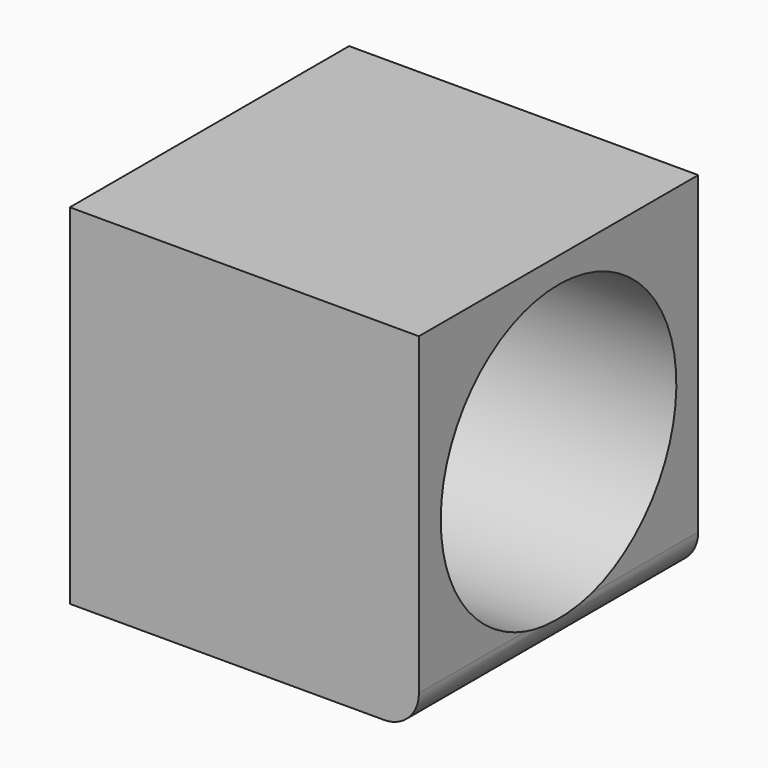
from build123d import *

# Parameters (mm, degrees)
F0_W        = 50
F0_H        = 50
F1_DEPTH    = 50
F2_R        = 21.0892085761
F4_DEPTH    = 50.001
F3_T1_DEPTH = 75


# Not quite as in the source:
# - a fillet or chamfer that OpenCascade refuses, or shapes differently, is made with other operations: its cross-section is extruded or revolved along the edge and cut away or added


with BuildPart() as f1:
    # F0 (on Top) → F1 (new body)
    with BuildSketch(Plane.XY):
        Rectangle(F0_W, F0_H)
    extrude(amount=F1_DEPTH)

    # F2 (on face) → F4 (cut, through all)
    with BuildSketch(Plane(origin=(-25, 0, 0), x_dir=(0, -1, 0), z_dir=(-1, 0, 0))):
        with Locations((0, 25.2627544105)):
            Circle(F2_R)
    extrude(amount=-F4_DEPTH, mode=Mode.SUBTRACT)

    # F3: fillet of radius 5 on 1 edges, made by hand

    # F3_s2 → F3_t1 (cut)
    with BuildSketch(Plane.XZ.offset(-37.5)):
        with BuildLine():
            ThreePointArc((25, 5), (23.5355339059, 1.4644660941), (20, 0))
            Line((20, 0), (25, 0))
            Line((25, 0), (25, 5))
        make_face()
    extrude(amount=F3_T1_DEPTH, mode=Mode.SUBTRACT)


solid = f1.part
